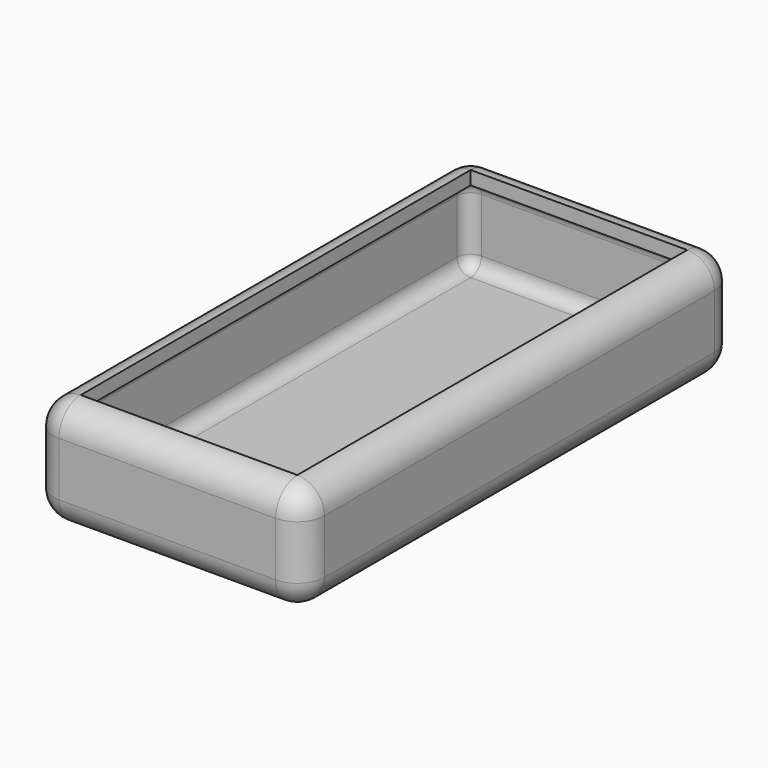
from build123d import *

# Parameters (mm, degrees)
F0_W     = 100
F0_H     = 20
F1_DEPTH = 50
F2_R     = 5
F3_T     = -2.5


# Not quite as in the source:
# - a shell that OpenCascade refuses in one call is made with other operations: the cavity is built on its own and cut out


with BuildPart() as f1:
    # F0 (on Right) → F1 (new body)
    with BuildSketch(Plane.YZ):
        Rectangle(F0_W, F0_H)
    extrude(amount=F1_DEPTH)

    # F2
    f2_edges = [f1.edges().sort_by_distance(p)[0] for p in [
        (25, -50, -10),
        (50, -50, 0),
        (0, -50, 0),
        (0, 0, -10),
        (50, 0, -10),
        (50, 50, 0),
        (0, 50, 0),
        (25, 50, -10),
        (25, 50, 10),
        (0, 0, 10),
        (25, -50, 10),
        (50, 0, 10),
    ]]
    fillet(f2_edges, radius=F2_R)

    # F3: a shell. OpenCascade refuses it in one call, so the cavity is built on its own and cut out:
    # the body offset inwards by the wall thickness, plus a prism from it out through each open face.
    f3_core = offset(f1.part, amount=F3_T, mode=Mode.PRIVATE)
    f3_exits = [f3_core.faces().sort_by_distance(p)[0] for p in [
        (25, 0, 7.5),
    ]]
    add(f3_core, mode=Mode.SUBTRACT)
    extrude(f3_exits, amount=-F3_T, mode=Mode.SUBTRACT)


solid = f1.part
